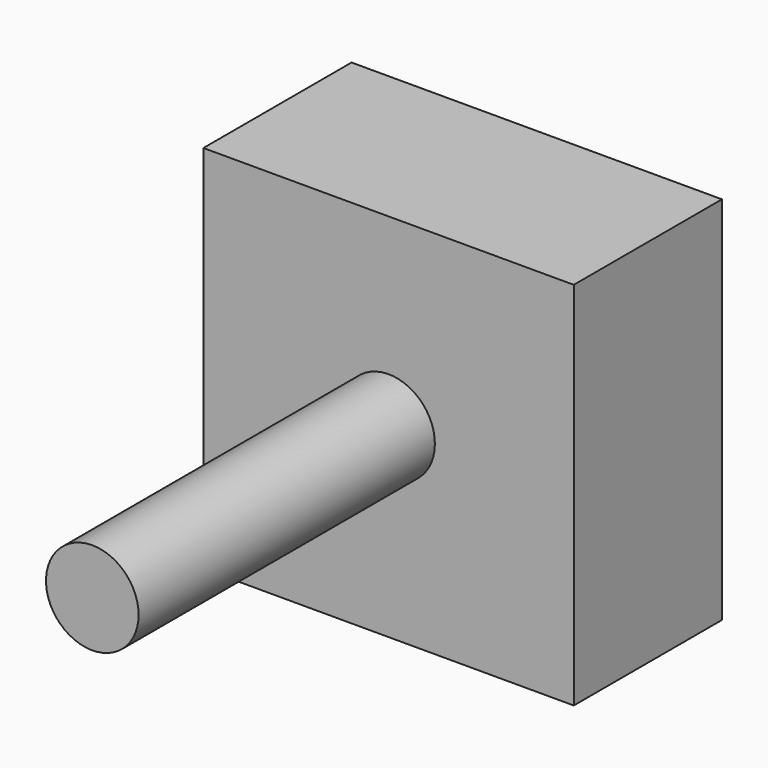
from build123d import *

# Parameters (mm, degrees)
F0_W     = 20
F0_H     = 50
F1_DEPTH = 60
F2_R     = 2.5
F3_DEPTH = 20
F4_DEPTH = 40
F5_DEPTH = 40
F6_DEPTH = 25
F7_DEPTH = 40
F8_DEPTH = 15


# Not quite as in the source:
# - a feature names something its author has since deleted; it is built from what else it names


with BuildPart() as f1:
    # F0 (on Top) → F1 (new body)
    with BuildSketch(Plane.XY):
        Rectangle(F0_W, F0_H)
    extrude(amount=F1_DEPTH)

    # F2 (on face) → F3 (cut)
    with BuildSketch(Plane.XZ.offset(25)):
        with Locations((0, 50)):
            Circle(F2_R)
    extrude(amount=-F3_DEPTH, mode=Mode.SUBTRACT)

    # F4 (add): a face of the model
    f4_faces = [f1.faces().sort_by_distance(p)[0] for p in [
        (0, 0, 0),
    ]]
    extrude(f4_faces, amount=-F4_DEPTH)

    # F5 (cut): a face of the model
    f5_faces = [f1.faces().sort_by_distance(p)[0] for p in [
        (0, 0, 0),
    ]]
    extrude(f5_faces, amount=-F5_DEPTH, mode=Mode.SUBTRACT)

    # F6 (cut): a face of the model
    f6_faces = [f1.faces().sort_by_distance(p)[0] for p in [
        (0, 25, 50),
    ]]
    extrude(f6_faces, amount=-F6_DEPTH, mode=Mode.SUBTRACT)

    # F7 (add): a face of the model
    f7_faces = [f1.faces().sort_by_distance(p)[0] for p in [
        (0, -5, 50),
    ]]
    extrude(f7_faces, amount=F7_DEPTH)

    # F8 (cut): a face of the model
    f8_faces = [f1.faces().sort_by_distance(p)[0] for p in [
        (0, 0, 50),
    ]]
    extrude(f8_faces, amount=-F8_DEPTH, mode=Mode.SUBTRACT)


solid = f1.part
